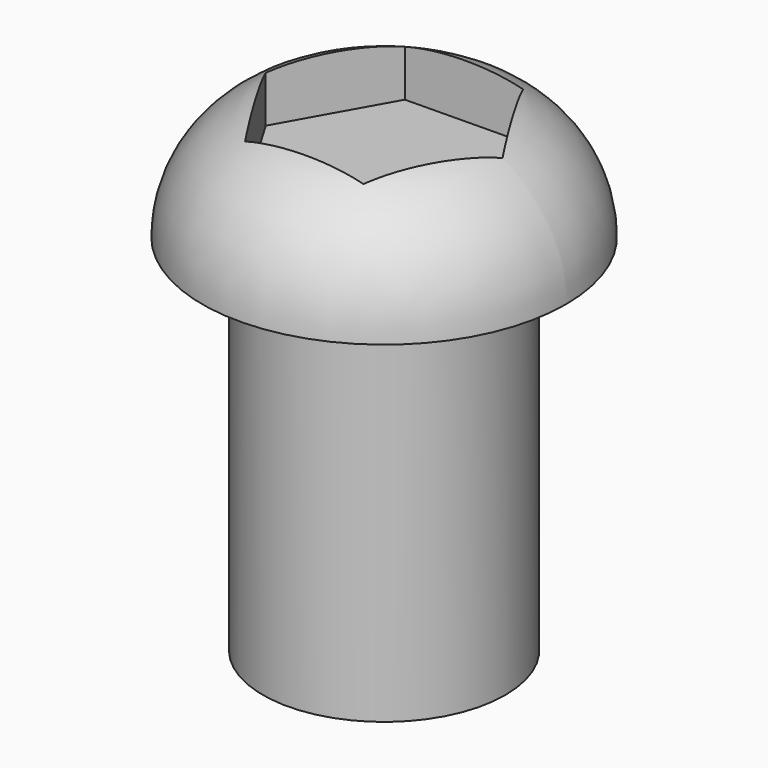
from build123d import *

# Parameters (mm, degrees)
F3_DEPTH = 3.175


# Not quite as in the source:
# - a fillet or chamfer that OpenCascade refuses, or shapes differently, is made with other operations: its cross-section is extruded or revolved along the edge and cut away or added


with BuildPart() as f1:
    # F0 (on Front) → F1 (revolve)
    with BuildSketch(Plane.XZ):
        Polygon((9.525, 17.8360301112), (0, 17.8360301112), (0, -7.5639698888), (6.35, -7.5639698888), (6.35, 11.4860301112), (9.525, 11.4860301112), align=None)
    revolve(axis=Axis((0, 0, 2.9950272292), (0, 0, -1)))

    # F2 (on face) → F3 (cut)
    with BuildSketch(Plane.XY.offset(17.8360301112)):
        Polygon((-3.001152127, -5.3557559125), (3.1376446132, -5.2769519389), (6.1387967402, 0.0788039736), (3.001152127, 5.3557559125), (-3.1376446132, 5.2769519389), (-6.1387967402, -0.0788039736), align=None)
    extrude(amount=-F3_DEPTH, mode=Mode.SUBTRACT)

    # F4: fillet of radius 6.35 on 1 edges, made by hand

    # F4_s1 → F4_t2 (revolve, cut)
    with BuildSketch(Plane.XZ):
        with BuildLine():
            ThreePointArc((3.175, 17.8360301112), (7.6651280605, 15.9761581718), (9.525, 11.4860301112))
            Line((9.525, 11.4860301112), (9.525, 17.8360301112))
            Line((9.525, 17.8360301112), (3.175, 17.8360301112))
        make_face()
    revolve(axis=Axis((0, 0, 17.8360301112), (0, 0, -1)), mode=Mode.SUBTRACT)


solid = f1.part
